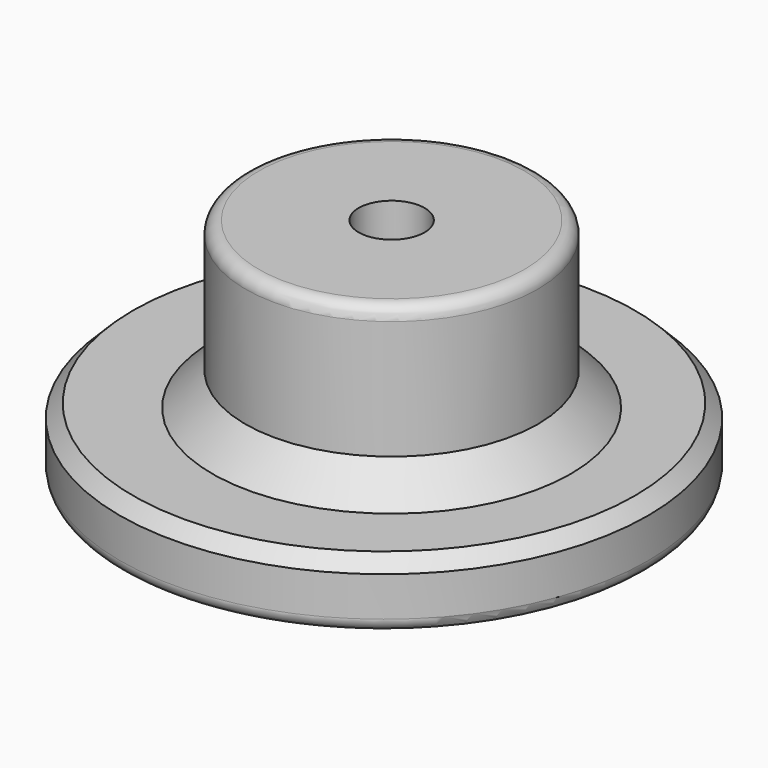
from build123d import *

# Parameters (mm, degrees)
F0_R     = 40
F1_DEPTH = 10
F2_SIZE  = 2
F3_R     = 22.145473903
F4_DEPTH = 25
F6_D     = 10
F7_R     = 2
F8_SIZE  = 5


with BuildPart() as f1:
    # F0 (on Top) → F1 (new body)
    with BuildSketch(Plane.XY):
        with Locations((-1.4435499907, 0.3608763218)):
            Circle(F0_R)
    extrude(amount=F1_DEPTH)

    # F2
    f2_edges = [f1.edges().sort_by_distance(p)[0] for p in [
        (-41.44355, 0.360876, 10),
    ]]
    chamfer(f2_edges, length=F2_SIZE)

    # F3 (on face) → F4 (join)
    with BuildSketch(Plane.XY.offset(10)):
        Circle(F3_R)
    extrude(amount=F4_DEPTH)

    # F6 (through all)
    with Locations(Plane.XY.offset(35)):
        with Locations((0, 0)):
            Hole(F6_D / 2)

    # F7
    f7_edges = [f1.edges().sort_by_distance(p)[0] for p in [
        (-41.44355, 0.360876, 0),
        (-22.145474, 0, 35),
        (-5, 0, 0),
    ]]
    fillet(f7_edges, radius=F7_R)

    # F8
    f8_edges = [f1.edges().sort_by_distance(p)[0] for p in [
        (22.145474, 0, 21.5),
        (-22.145474, 0, 33),
        (-22.145474, 0, 10),
    ]]
    chamfer(f8_edges, length=F8_SIZE)


solid = f1.part
